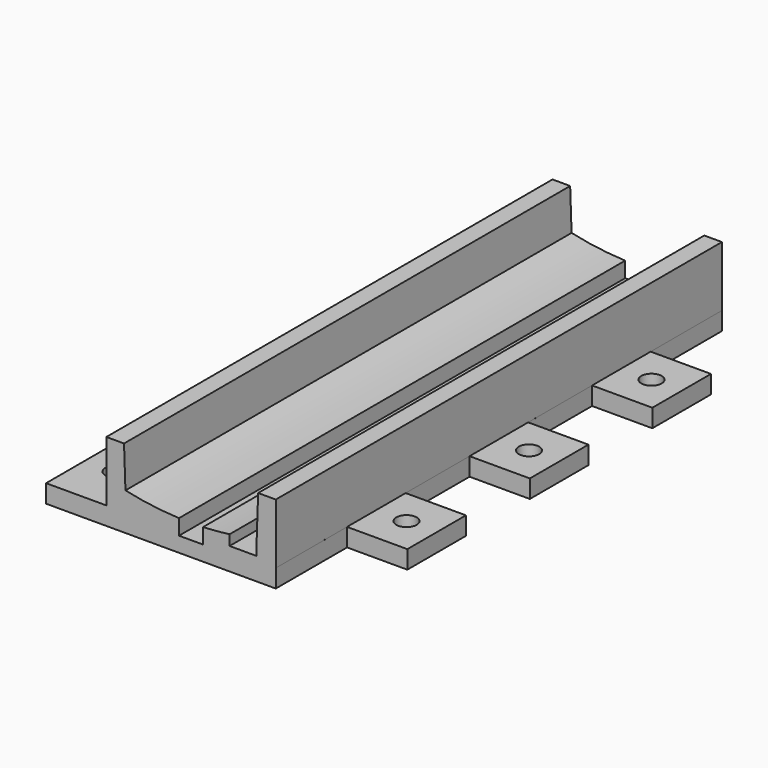
from build123d import *

# Parameters (mm, degrees)
F1_DEPTH = 185
F3_DEPTH = 30
F2_W     = 10
F2_H     = 12.7
F2_W_2   = 20
F2_H_2   = 29.6450595204
F2_H_3   = 26.5
F2_H_4   = 30.8181657076
F4_DEPTH = 25
F5_D     = 6.7564


# Not quite as in the source:
# - a feature names something its author has since deleted; it is built from what else it names


with BuildPart() as f1:
    # F0 (on Front) → F1 (new body)
    with BuildSketch(Plane.XZ):
        with BuildLine():
            Line((-28.0998, -84.153), (-28.0998, -96.0750292217))
            ThreePointArc((-28.0998, -96.0750292217), (-24.948943425, -96.9410141373), (-21.7715, -97.7036938286))
            Line((-21.7715, -97.7036938286), (-22.2458, -84.153))
            Line((-22.2458, -84.153), (-28.0998, -84.153))
        make_face()
        with BuildLine():
            ThreePointArc((-21.7715, -97.7036938286), (-24.948943425, -96.9410141373), (-28.0998, -96.0750292217))
            Line((-28.0998, -96.0750292217), (-28.0998, -104.153))
            Line((-28.0998, -104.153), (-48.0998, -104.153))
            Line((-48.0998, -104.153), (-48.0998, -110.153))
            Line((-48.0998, -110.153), (0, -110.153))
            Line((0, -110.153), (48.0998, -110.153))
            Line((48.0998, -110.153), (48.0998, -104.153))
            Line((48.0998, -104.153), (28.0998, -104.153))
            Line((28.0998, -104.153), (28.0998, -96.0750292217))
            ThreePointArc((28.0998, -96.0750292217), (24.948943425, -96.9410141373), (21.7715, -97.7036938286))
            Line((21.7715, -97.7036938286), (21.7715, -102.7036938286))
            Line((21.7715, -102.7036938286), (12.7715, -102.7036938286))
            Line((12.7715, -102.7036938286), (12.7715, -99.2819157135))
            ThreePointArc((12.7715, -99.2819157135), (8.3938675756, -99.747446018), (4, -100.0200479904))
            Line((4, -100.0200479904), (4, -105.1526938286))
            Line((4, -105.1526938286), (-4, -105.1526938286))
            Line((-4, -105.1526938286), (-4, -100.0200479904))
            ThreePointArc((-4, -100.0200479904), (-12.9376940454, -99.2603952883), (-21.7715, -97.7036938286))
        make_face()
        with BuildLine():
            ThreePointArc((21.7715, -97.7036938286), (24.948943425, -96.9410141373), (28.0998, -96.0750292217))
            Line((28.0998, -96.0750292217), (28.0998, -84.153))
            Line((28.0998, -84.153), (22.2458, -84.153))
            Line((22.2458, -84.153), (21.7715, -97.7036938286))
        make_face()
        with BuildLine():
            Line((21.7715, -102.7036938286), (21.7715, -97.7036938286))
            ThreePointArc((21.7715, -97.7036938286), (17.289517296, -98.5955505673), (12.7715, -99.2819157135))
            Line((12.7715, -99.2819157135), (12.7715, -102.7036938286))
            Line((12.7715, -102.7036938286), (21.7715, -102.7036938286))
        make_face()
    extrude(amount=-F1_DEPTH)

    # F0 (on Front) → F3 (cut)
    with BuildSketch(Plane.XZ):
        with BuildLine():
            Line((21.7715, -102.7036938286), (21.7715, -97.7036938286))
            ThreePointArc((21.7715, -97.7036938286), (17.289517296, -98.5955505673), (12.7715, -99.2819157135))
            Line((12.7715, -99.2819157135), (12.7715, -102.7036938286))
            Line((12.7715, -102.7036938286), (21.7715, -102.7036938286))
        make_face()
    extrude(amount=-F3_DEPTH, mode=Mode.SUBTRACT)

    # F2 (on face) → F4 (cut)
    with BuildSketch(Plane.XY.offset(-104.153)):
        Polygon((-48.0998, 29), (-38.0998, 29), (-38.0998, 41.7), (-38.0998, 54.4), (-48.0998, 54.4), align=None)
        with Locations((-33.0998, 35.35)):
            Rectangle(F2_W, F2_H)
        Polygon((-48.0998, 105.2), (-48.0998, 79.8), (-38.0998, 79.8), (-38.0998, 92.5), (-38.0998, 105.2), align=None)
        with Locations((-33.0998, 86.15)):
            Rectangle(F2_W, F2_H)
        Polygon((-48.0998, 156), (-48.0998, 130.6), (-38.0998, 130.6), (-38.0998, 143.3), (-38.0998, 156), align=None)
        with Locations((-33.0998, 136.95)):
            Rectangle(F2_W, F2_H)
        with Locations((-33.0998, 48.05)):
            Rectangle(F2_W, F2_H)
        with Locations((-33.0998, 98.85)):
            Rectangle(F2_W, F2_H)
        with Locations((-33.0998, 149.65)):
            Rectangle(F2_W, F2_H)
        with Locations((38.1002, 14.7274702398)):
            Rectangle(F2_W_2, F2_H_2)
        with Locations((38.1002, 67.1)):
            Rectangle(F2_W_2, F2_H_3)
        with Locations((38.1002, 117.9)):
            Rectangle(F2_W_2, F2_H_3)
        with Locations((38.1002, 170.8590828538)):
            Rectangle(F2_W_2, F2_H_4)
    extrude(amount=-F4_DEPTH, mode=Mode.SUBTRACT)

    # F5 (through all)
    with Locations(Plane.XY.offset(-104.153)):
        with Locations((-38.0998, 67.1), (-38.0998, 16.3), (-38.0998, 117.9), (-38.0998, 168.7), (38.1002, 92.5), (38.1002, 143.3), (38.1002, 41.7)):
            Hole(F5_D / 2)


solid = f1.part
